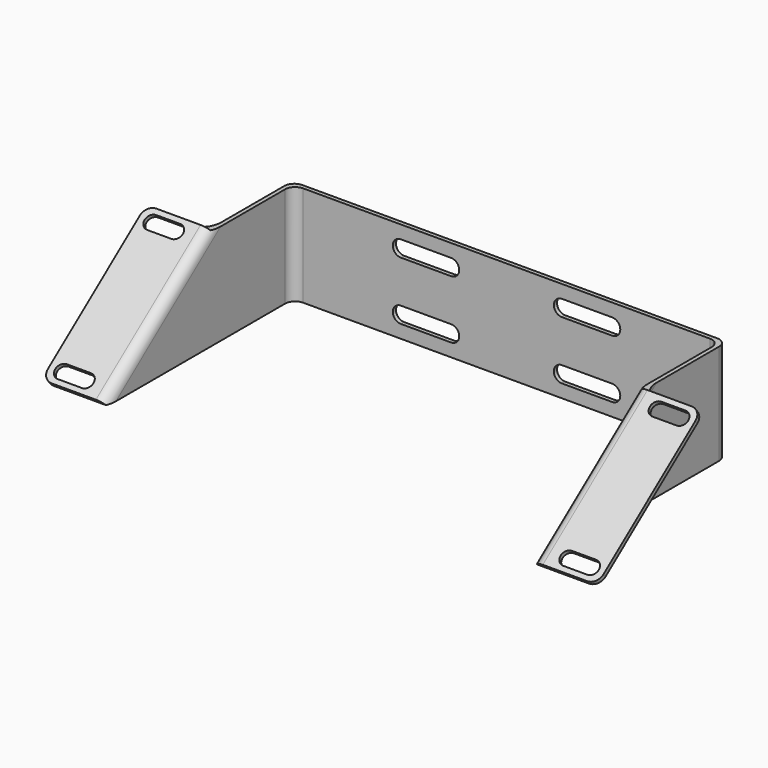
from build123d import *

# Parameters (mm, degrees)
F0_W     = 216
F0_H     = 50
F1_DEPTH = 2
F3_DEPTH = 2
F4_W     = 32
F4_H     = 82.0060973343
F5_DEPTH = 2
F7_DEPTH = 2
F8_W     = 32
F8_H     = 82.0060973343
F9_DEPTH = 2
F10_R    = 5


# Not quite as in the source:
# - a feature names something its author has since deleted; it is built from what else it names


with BuildPart() as f1:
    # F0 (on Front) → F1 (new body)
    with BuildSketch(Plane.XZ):
        Rectangle(F0_W, F0_H)
        with BuildLine():
            ThreePointArc((-27.5, -10.5), (-24.6715728753, -11.6715728753), (-23.5, -14.5))
            ThreePointArc((-23.5, -14.5), (-24.6715728753, -17.3284271247), (-27.5, -18.5))
            Line((-27.5, -18.5), (-52.5, -18.5))
            ThreePointArc((-52.5, -18.5), (-56.5, -14.5), (-52.5, -10.5))
            Line((-52.5, -10.5), (-27.5, -10.5))
        make_face(mode=Mode.SUBTRACT)
        with BuildLine():
            ThreePointArc((27.5, -18.5), (23.5, -14.5), (27.5, -10.5))
            Line((27.5, -10.5), (52.5, -10.5))
            ThreePointArc((52.5, -10.5), (55.3284271247, -11.6715728753), (56.5, -14.5))
            ThreePointArc((56.5, -14.5), (55.3284271247, -17.3284271247), (52.5, -18.5))
            Line((52.5, -18.5), (27.5, -18.5))
        make_face(mode=Mode.SUBTRACT)
        with BuildLine():
            ThreePointArc((-52.5, 10.5), (-56.5, 14.5), (-52.5, 18.5))
            Line((-52.5, 18.5), (-27.5, 18.5))
            ThreePointArc((-27.5, 18.5), (-24.6715728753, 17.3284271247), (-23.5, 14.5))
            ThreePointArc((-23.5, 14.5), (-24.6715728753, 11.6715728753), (-27.5, 10.5))
            Line((-27.5, 10.5), (-52.5, 10.5))
        make_face(mode=Mode.SUBTRACT)
        with BuildLine():
            ThreePointArc((27.5, 10.5), (23.5, 14.5), (27.5, 18.5))
            Line((27.5, 18.5), (52.5, 18.5))
            ThreePointArc((52.5, 18.5), (55.3284271247, 17.3284271247), (56.5, 14.5))
            ThreePointArc((56.5, 14.5), (55.3284271247, 11.6715728753), (52.5, 10.5))
            Line((52.5, 10.5), (27.5, 10.5))
        make_face(mode=Mode.SUBTRACT)
    extrude(amount=-F1_DEPTH)

    # F2 (on face) → F3 (join)
    with BuildSketch(Plane(origin=(-108, 0, 0), x_dir=(0, -1, 0), z_dir=(-1, 0, 0))):
        Polygon((0, 25), (0, -25), (115, -25), (50, 25), align=None)
    extrude(amount=-F3_DEPTH)

    # F4 (on face) → F5 (join)
    with BuildSketch(Plane(origin=(0, -30.6691449814, 39.8698884758), x_dir=(1, 0, 0), z_dir=(0, -0.6097107608, 0.7926239891))):
        with Locations((-122, -65.3914791011)):
            Rectangle(F4_W, F4_H)
        with BuildLine():
            ThreePointArc((-119.5, -96.8914791011), (-117.0251262658, -97.916605367), (-116, -100.3914791011))
            ThreePointArc((-116, -100.3914791011), (-117.0251262658, -102.8663528353), (-119.5, -103.8914791011))
            Line((-119.5, -103.8914791011), (-131.5, -103.8914791011))
            ThreePointArc((-131.5, -103.8914791011), (-135, -100.3914791011), (-131.5, -96.8914791011))
            Line((-131.5, -96.8914791011), (-119.5, -96.8914791011))
        make_face(mode=Mode.SUBTRACT)
        with BuildLine():
            ThreePointArc((-131.5, -33.8914791011), (-135, -30.3914791011), (-131.5, -26.8914791011))
            Line((-131.5, -26.8914791011), (-119.5, -26.8914791011))
            ThreePointArc((-119.5, -26.8914791011), (-117.0251262658, -27.916605367), (-116, -30.3914791011))
            ThreePointArc((-116, -30.3914791011), (-117.0251262658, -32.8663528353), (-119.5, -33.8914791011))
            Line((-119.5, -33.8914791011), (-131.5, -33.8914791011))
        make_face(mode=Mode.SUBTRACT)
    extrude(amount=F5_DEPTH)

    # F6 (on face) → F7 (join)
    with BuildSketch(Plane.YZ.offset(108)):
        Polygon((0, -25), (0, 25), (-50, 25), (-115, -25), align=None)
    extrude(amount=-F7_DEPTH)

    # F8 (on face) → F9 (join)
    with BuildSketch(Plane(origin=(0, -30.6691449814, 39.8698884758), x_dir=(1, 0, 0), z_dir=(0, -0.6097107608, 0.7926239891))):
        with Locations((122, -65.3914791011)):
            Rectangle(F8_W, F8_H)
        with BuildLine():
            ThreePointArc((131.5, -96.8914791011), (133.9748737342, -97.916605367), (135, -100.3914791011))
            ThreePointArc((135, -100.3914791011), (133.9748737342, -102.8663528353), (131.5, -103.8914791011))
            Line((131.5, -103.8914791011), (119.5, -103.8914791011))
            ThreePointArc((119.5, -103.8914791011), (116, -100.3914791011), (119.5, -96.8914791011))
            Line((119.5, -96.8914791011), (131.5, -96.8914791011))
        make_face(mode=Mode.SUBTRACT)
        with BuildLine():
            ThreePointArc((119.5, -33.8914791011), (116, -30.3914791011), (119.5, -26.8914791011))
            Line((119.5, -26.8914791011), (131.5, -26.8914791011))
            ThreePointArc((131.5, -26.8914791011), (133.9748737342, -27.916605367), (135, -30.3914791011))
            ThreePointArc((135, -30.3914791011), (133.9748737342, -32.8663528353), (131.5, -33.8914791011))
            Line((131.5, -33.8914791011), (119.5, -33.8914791011))
        make_face(mode=Mode.SUBTRACT)
    extrude(amount=F9_DEPTH)

    # F10
    f10_edges = [f1.edges().sort_by_distance(p)[0] for p in [
        (-106, -83.719422, 1.585248),
        (-108, -82.5, 0),
        (-108, 2, 0),
        (-106, 0, 0),
        (106, 0, 0),
        (108, 2, 0),
        (108, -82.5, 0),
        (-138, -115.609711, -24.207376),
        (-138, -50.609711, 25.792624),
        (106, -83.719422, 1.585248),
        (138, -50.609711, 25.792624),
        (138, -115.609711, -24.207376),
    ]]
    fillet(f10_edges, radius=F10_R)


solid = f1.part
